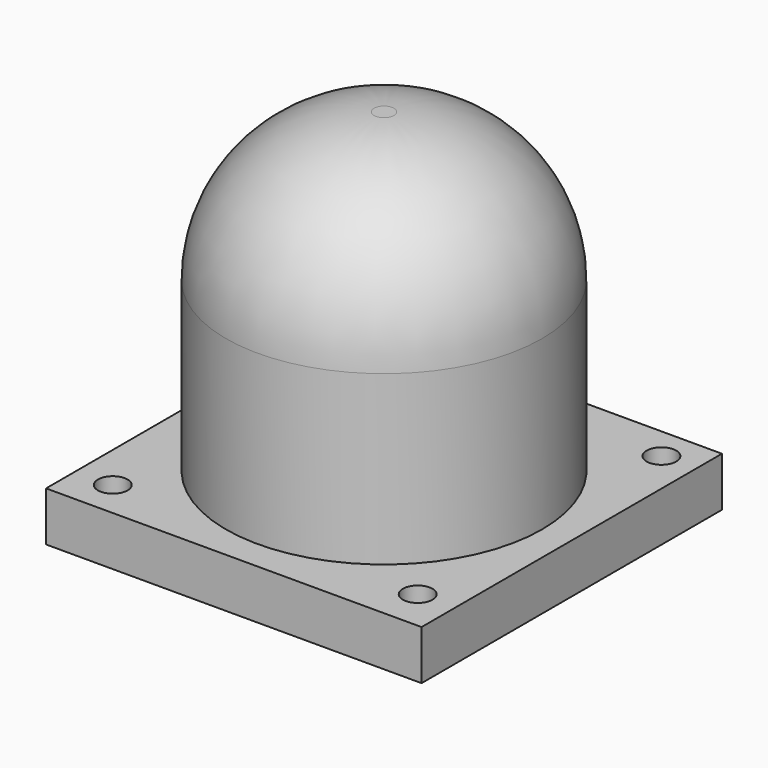
from build123d import *

# Parameters (mm, degrees)
F0_R     = 16
F1_DEPTH = 37
F0_W     = 38
F0_H     = 38
F0_R_2   = 1.5
F2_DEPTH = 5
F3_R     = 15
F4_T     = -2.5


with BuildPart() as f1:
    # F0 (on Top) → F1 (new body)
    with BuildSketch(Plane.XY):
        with Locations((19, 19)):
            Circle(F0_R)
    extrude(amount=F1_DEPTH)

    # F3
    f3_edges = [f1.edges().sort_by_distance(p)[0] for p in [
        (3, 19, 37),
    ]]
    fillet(f3_edges, radius=F3_R)

    # F4
    f4_openings = [f1.faces().sort_by_distance(p)[0] for p in [
        (19, 19, 0),
    ]]
    offset(amount=F4_T, openings=f4_openings)


with BuildPart() as f2:
    # F0 (on Top) → F2 (new body)
    with BuildSketch(Plane.XY):
        with Locations((19, 19)):
            Rectangle(F0_W, F0_H)
        with Locations((3.75, 3.75)):
            Circle(F0_R_2, mode=Mode.SUBTRACT)
        with Locations((34.25, 4.1987560689)):
            Circle(F0_R_2, mode=Mode.SUBTRACT)
        with Locations((4.0231071115, 34.25)):
            Circle(F0_R_2, mode=Mode.SUBTRACT)
        with Locations((19, 19)):
            Circle(F0_R, mode=Mode.SUBTRACT)
        with Locations((34.5231071115, 34.6987560689)):
            Circle(F0_R_2, mode=Mode.SUBTRACT)
    extrude(amount=F2_DEPTH)


solid = Compound([f1.part, f2.part])
